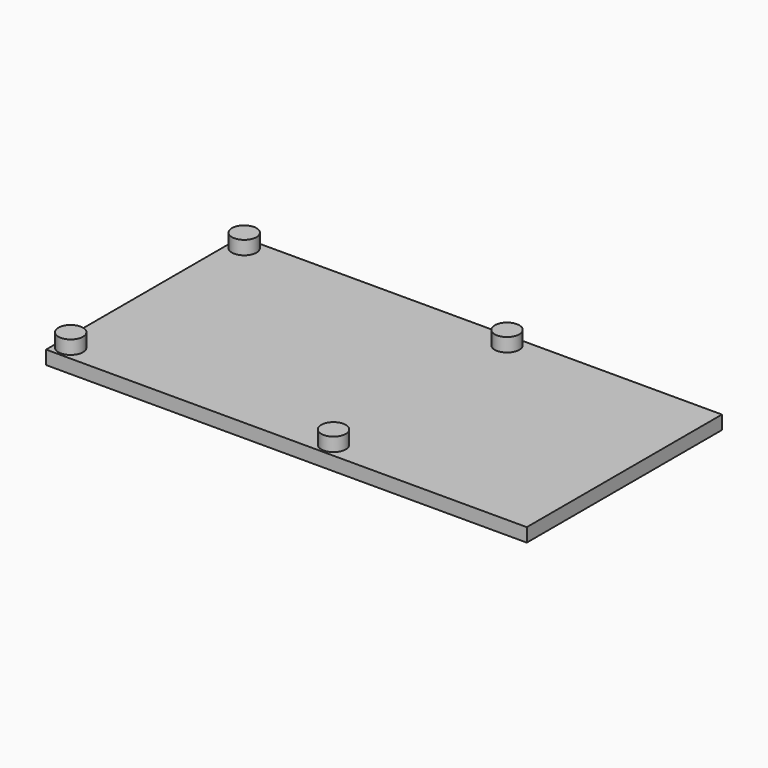
from build123d import *

# Parameters (mm, degrees)
F0_R     = 2.25
F1_DEPTH = 5
F0_W     = 53.1
F0_H     = 44.7
F2_DEPTH = 2.5
F6_DEPTH = 35


# Not quite as in the source:
# - the program builds the solid bodies; features that only make, move or delete a surface that nothing else refers to are left out


with BuildPart() as f1:
    # F0 (on Top) → F1 (new body)
    with BuildSketch(Plane.XY):
        with Locations((24.1313669831, 19.8986493051)):
            Circle(F0_R)
    extrude(amount=F1_DEPTH)


with BuildPart() as f1b:
    # F0 (on Top) → F1, piece 2 (new body)
    with BuildSketch(Plane.XY):
        with Locations((-24.0537095815, 19.9159570038)):
            Circle(F0_R)
    extrude(amount=F1_DEPTH)


with BuildPart() as f1c:
    # F0 (on Top) → F1, piece 3 (new body)
    with BuildSketch(Plane.XY):
        with Locations((-24.1623297334, -19.694061164)):
            Circle(F0_R)
    extrude(amount=F1_DEPTH)


with BuildPart() as f1d:
    # F0 (on Top) → F1, piece 4 (new body)
    with BuildSketch(Plane.XY):
        with Locations((24.0227468312, -19.7113688628)):
            Circle(F0_R)
    extrude(amount=F1_DEPTH)


with BuildPart() as f2:
    # F0 (on Top) → F2 (new body)
    with BuildSketch(Plane.XY):
        Rectangle(F0_W, F0_H)
        with Locations((-24.1623297334, -19.694061164)):
            Circle(F0_R, mode=Mode.SUBTRACT)
        with Locations((24.0227468312, -19.7113688628)):
            Circle(F0_R, mode=Mode.SUBTRACT)
        with Locations((-24.0537095815, 19.9159570038)):
            Circle(F0_R, mode=Mode.SUBTRACT)
        with Locations((24.1313669831, 19.8986493051)):
            Circle(F0_R, mode=Mode.SUBTRACT)
    extrude(amount=F2_DEPTH)

    # F6 (add): a face of the model
    f6_faces = [f2.faces().sort_by_distance(p)[0] for p in [
        (26.55, 0, 1.25),
    ]]
    extrude(f6_faces, amount=F6_DEPTH)


solid = Compound([f1.part, f1b.part, f1c.part, f1d.part, f2.part])
